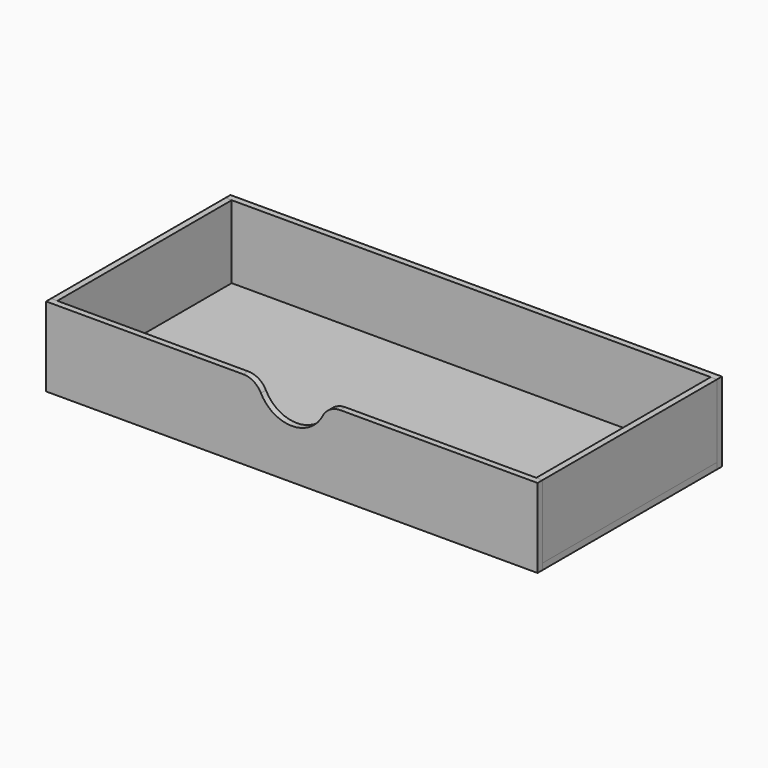
from build123d import *

# Parameters (mm, degrees)
F1_W      = 248
F1_H      = 40
F2_DEPTH  = 3.15
F3_R      = 17.5
F4_DEPTH  = 25
F5_R      = 10
F6_W      = 110
F6_H      = 36.85
F7_DEPTH  = 3.15
F9_W      = 248
F9_H      = 40
F10_DEPTH = 3.15
F11_W     = 248
F11_H     = 110
F12_DEPTH = 3.15


with BuildPart() as f2:
    # F1 (on Front) → F2 (new body)
    with BuildSketch(Plane.XZ):
        with Locations((124, 20)):
            Rectangle(F1_W, F1_H)
    extrude(amount=F2_DEPTH)

    # F3 (on face) → F4 (cut)
    with BuildSketch(Plane.XZ.offset(3.15)):
        with Locations((124, 42.5)):
            Circle(F3_R)
    extrude(amount=-F4_DEPTH, mode=Mode.SUBTRACT)

    # F5
    f5_edges = [f2.edges().sort_by_distance(p)[0] for p in [
        (106.679492, -1.575, 40),
        (141.320508, -1.575, 40),
    ]]
    fillet(f5_edges, radius=F5_R)


with BuildPart() as f7:
    # F6 (on face) → F7 (new body)
    with BuildSketch(Plane.YZ.offset(248)):
        with Locations((55, 21.575)):
            Rectangle(F6_W, F6_H)
    extrude(amount=-F7_DEPTH)


with BuildPart() as f8_1:
    # F8: copy of F7
    add(f7.part.moved(Location((-244.85, 0, 0))))


with BuildPart() as f10:
    # F9 (on face) → F10 (new body)
    with BuildSketch(Plane(origin=(0, 110, 0), x_dir=(-1, 0, 0), z_dir=(0, 1, 0))):
        with Locations((-124, 20)):
            Rectangle(F9_W, F9_H)
    extrude(amount=F10_DEPTH)


with BuildPart() as f12:
    # F11 (on face) → F12 (new body)
    with BuildSketch(Plane(origin=(0, 0, 3.15), x_dir=(1, 0, 0), z_dir=(0, 0, -1))):
        with Locations((124, -55)):
            Rectangle(F11_W, F11_H)
    extrude(amount=F12_DEPTH)


solid = Compound([f2.part, f7.part, f8_1.part, f10.part, f12.part])
